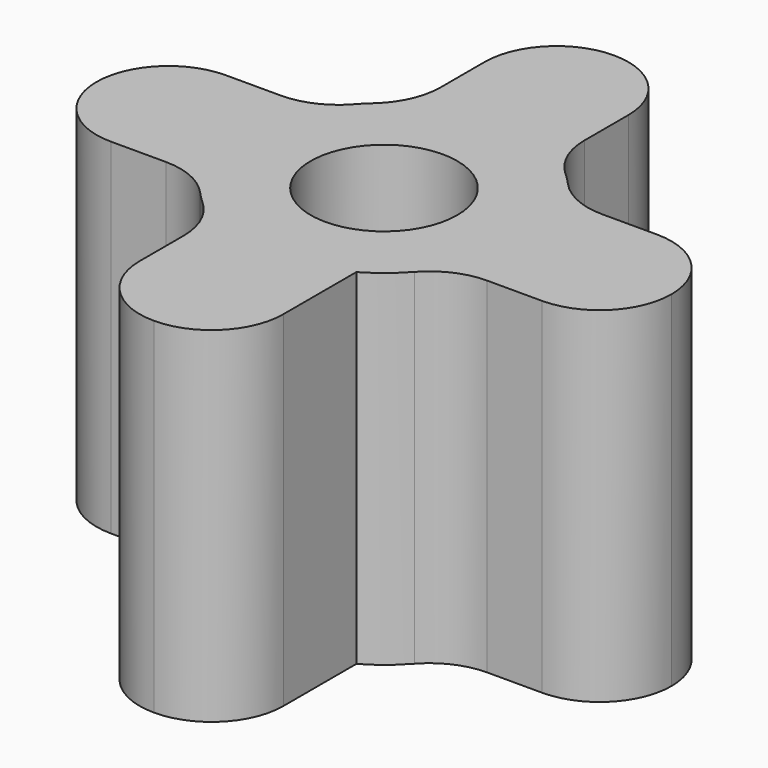
from build123d import *

# Parameters (mm, degrees)
F0_R     = 5
F0_R_2   = 2.55
F1_DEPTH = 12
F3_DEPTH = 12
F4_R     = 2.49999


# Not quite as in the source:
# - a fillet or chamfer is up to 0.001 mm smaller than in the source, because OpenCascade refuses the exact size


with BuildPart() as f1:
    # F0 (on Top) → F1 (new body)
    with BuildSketch(Plane.XY):
        Circle(F0_R)
        Circle(F0_R_2, mode=Mode.SUBTRACT)
    extrude(amount=F1_DEPTH)

    # F2 (on face) → F3 (join)
    with BuildSketch(Plane.XY.offset(12)):
        with BuildLine():
            Line((-2.5, 10), (-2.5, 4.3301270189))
            ThreePointArc((-2.5, 4.3301270189), (0, 5), (2.5, 4.3301270189))
            Line((2.5, 4.3301270189), (2.5, 10))
            Line((2.5, 10), (-2.5, 10))
        make_face()
        with BuildLine():
            Line((10, 2.5), (4.3301270189, 2.5))
            ThreePointArc((4.3301270189, 2.5), (4.8296291314, 1.2940952255), (5, 0))
            ThreePointArc((5, 0), (4.8296291314, -1.2940952255), (4.3301270189, -2.5))
            Line((4.3301270189, -2.5), (10, -2.5))
            Line((10, -2.5), (10, 2.5))
        make_face()
        with BuildLine():
            ThreePointArc((2.5, -4.3301270189), (0, -5), (-2.5, -4.3301270189))
            Line((-2.5, -4.3301270189), (-2.5, -10))
            Line((-2.5, -10), (2.5, -10))
            Line((2.5, -10), (2.5, -4.3301270189))
        make_face()
        with BuildLine():
            ThreePointArc((-4.3301270189, -2.5), (-5, 0), (-4.3301270189, 2.5))
            Line((-4.3301270189, 2.5), (-10, 2.5))
            Line((-10, 2.5), (-10, -2.5))
            Line((-10, -2.5), (-4.3301270189, -2.5))
        make_face()
    extrude(amount=-F3_DEPTH)

    # F4 (radius 2.5 in the source; OpenCascade refuses exactly that, so slightly less here)
    f4_edges = [f1.edges().sort_by_distance(p)[0] for p in [
        (2.5, -10, 6),
        (10, -2.5, 6),
        (-10, -2.5, 6),
        (-2.5, -10, 6),
        (-10, 2.5, 6),
        (-2.5, 10, 6),
        (10, 2.5, 6),
        (2.5, 10, 6),
        (2.5, 4.330127, 6),
        (4.330127, 2.5, 6),
        (4.330127, -2.5, 6),
        (-2.5, 4.330127, 6),
        (-4.330127, 2.5, 6),
        (-2.5, -4.330127, 6),
        (-4.330127, -2.5, 6),
    ]]
    fillet(f4_edges, radius=F4_R)


solid = f1.part
